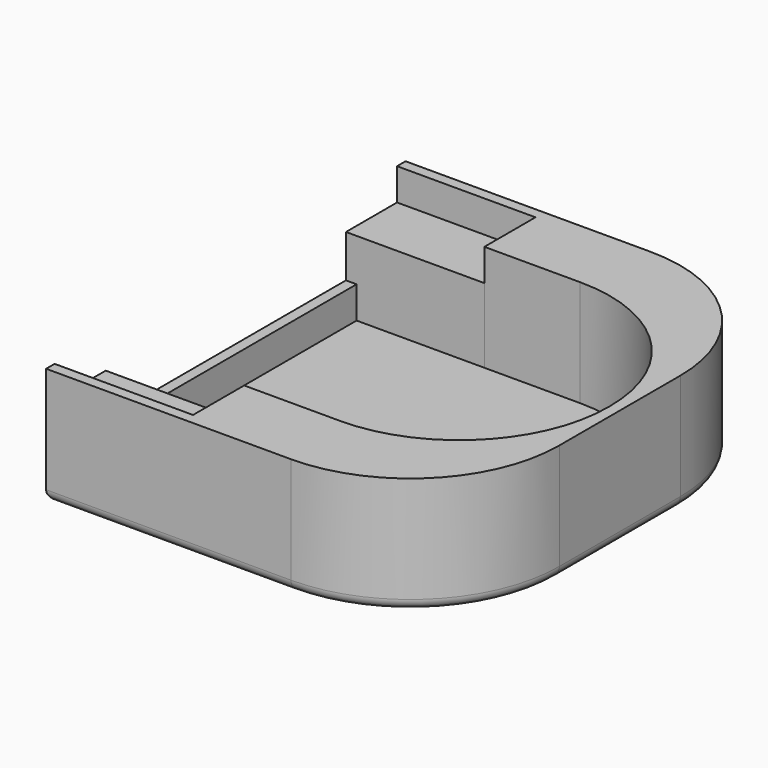
from build123d import *

# Parameters (mm, degrees)
F0_W     = 1
F0_H     = 28.2
F1_DEPTH = 3
F0_H_2   = 6
F0_W_2   = 12
F2_DEPTH = 7
F0_W_3   = 23
F3_DEPTH = 10
F4_DEPTH = 1
F5_R     = 14
F5_2_R   = 14
F6_R     = 0.99999


# Not quite as in the source:
# - a fillet or chamfer is up to 0.001 mm smaller than in the source, because OpenCascade refuses the exact size


with BuildPart() as f1:
    # F0 (on Top) → F1 (new body)
    with BuildSketch(Plane.XY):
        with Locations((-18, 0)):
            Rectangle(F0_W, F0_H)
    extrude(amount=F1_DEPTH)


with BuildPart() as f2:
    # F0 (on Top) → F2 (new body)
    with BuildSketch(Plane.XY):
        with Locations((-18, 17.1)):
            Rectangle(F0_W, F0_H_2)
        with Locations((-11.5, 17.1)):
            Rectangle(F0_W_2, F0_H_2)
    extrude(amount=F2_DEPTH)


with BuildPart() as f2b:
    # F0 (on Top) → F2, piece 2 (new body)
    with BuildSketch(Plane.XY):
        with Locations((-18, -17.1)):
            Rectangle(F0_W, F0_H_2)
        with Locations((-11.5, -17.1)):
            Rectangle(F0_W_2, F0_H_2)
    extrude(amount=F2_DEPTH)


with BuildPart() as f3:
    # F0 (on Top) → F3 (new body)
    with BuildSketch(Plane.XY):
        Polygon((17.5, -14.1), (17.5, -20.1), (-5.5, -20.1), (-17.5, -20.1), (-18.5, -20.1), (-18.5, -21.1), (18.5, -21.1), (18.5, 21.1), (-18.5, 21.1), (-18.5, 20.1), (-17.5, 20.1), (-5.5, 20.1), (17.5, 20.1), (17.5, 14.1), align=None)
        with Locations((6, 17.1)):
            Rectangle(F0_W_3, F0_H_2)
        with Locations((6, -17.1)):
            Rectangle(F0_W_3, F0_H_2)
    extrude(amount=F3_DEPTH)

    # F5
    f5_edges = [f3.edges().sort_by_distance(p)[0] for p in [
        (17.5, 14.1, 5),
        (17.5, -14.1, 5),
        (18.5, 21.1, 5),
        (18.5, -21.1, 5),
    ]]
    fillet(f5_edges, radius=F5_R)


with BuildPart() as f4:
    # F0 (on Top) → F4 (new body)
    with BuildSketch(Plane.XY):
        Polygon((-5.5, -14.1), (17.5, -14.1), (17.5, 14.1), (-5.5, 14.1), (-17.5, 14.1), (-17.5, -14.1), align=None)
        with Locations((-18, 17.1)):
            Rectangle(F0_W, F0_H_2)
        Polygon((17.5, -14.1), (17.5, -20.1), (-5.5, -20.1), (-17.5, -20.1), (-18.5, -20.1), (-18.5, -21.1), (18.5, -21.1), (18.5, 21.1), (-18.5, 21.1), (-18.5, 20.1), (-17.5, 20.1), (-5.5, 20.1), (17.5, 20.1), (17.5, 14.1), align=None)
        with Locations((-11.5, 17.1)):
            Rectangle(F0_W_2, F0_H_2)
        with Locations((6, 17.1)):
            Rectangle(F0_W_3, F0_H_2)
        with Locations((-18, 0)):
            Rectangle(F0_W, F0_H)
        with Locations((-18, -17.1)):
            Rectangle(F0_W, F0_H_2)
        with Locations((-11.5, -17.1)):
            Rectangle(F0_W_2, F0_H_2)
        with Locations((6, -17.1)):
            Rectangle(F0_W_3, F0_H_2)
    extrude(amount=-F4_DEPTH)

    # F5#2
    f5_2_edges = [f4.edges().sort_by_distance(p)[0] for p in [
        (18.5, 21.1, -0.5),
        (18.5, -21.1, -0.5),
    ]]
    fillet(f5_2_edges, radius=F5_2_R)

    # F6 (radius 1 in the source; OpenCascade refuses exactly that, so slightly less here)
    f6_edges = [f4.edges().sort_by_distance(p)[0] for p in [
        (-7, -21.1, -1),
        (-18.5, 0, -1),
    ]]
    fillet(f6_edges, radius=F6_R)


solid = Compound([f1.part, f2.part, f2b.part, f3.part, f4.part])
